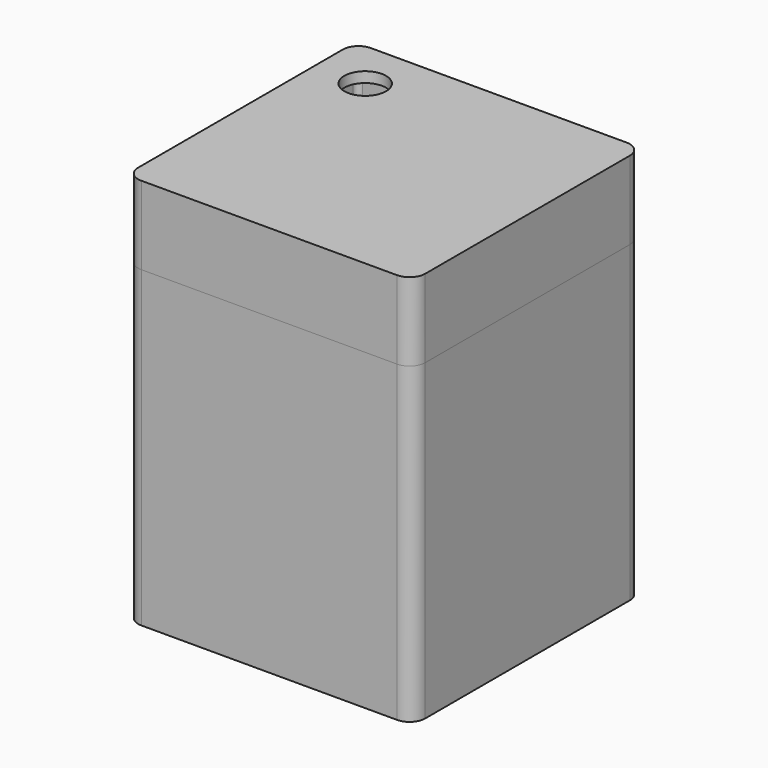
from build123d import *

# Parameters (mm, degrees)
F0_W      = 55
F0_H      = 55
F1_DEPTH  = 15
F2_R      = 3
F3_T      = -2
F4_R      = 4
F5_DEPTH  = 25
F6_DEPTH  = 60
F8_DEPTH  = 3
F9_W      = 5
F9_H      = 5
F10_DEPTH = 5
F11_R     = 2
F13_D     = 1.8
F13_DEPTH = 5
F13_TIP   = 0.5407745571


# Not quite as in the source:
# - a feature names something its author has since deleted; it is built from what else it names


with BuildPart() as f1:
    # F0 (on Top) → F1 (new body)
    with BuildSketch(Plane.XY):
        Rectangle(F0_W, F0_H)
    extrude(amount=F1_DEPTH)

    # F2
    f2_edges = [f1.edges().sort_by_distance(p)[0] for p in [
        (-27.5, 27.5, 7.5),
        (-27.5, -27.5, 7.5),
        (27.5, -27.5, 7.5),
        (27.5, 27.5, 7.5),
    ]]
    fillet(f2_edges, radius=F2_R)

    # F3
    f3_openings = [f1.faces().sort_by_distance(p)[0] for p in [
        (0, 0, 0),
    ]]
    offset(amount=F3_T, openings=f3_openings)

    # F4 (on face) → F5 (cut)
    with BuildSketch(Plane.XY.offset(15)):
        with Locations((-18, 18)):
            Circle(F4_R)
    extrude(amount=-F5_DEPTH, mode=Mode.SUBTRACT)


with BuildPart() as f6:
    # F6 (new): a face of the model
    f6_faces = [f1.part.faces().sort_by_distance(p)[0] for p in [
        (0, -26.7221825407, 0),
    ]]
    extrude(f6_faces, amount=F6_DEPTH)

    # F7 (on face) → F8 (cut)
    with BuildSketch(Plane(origin=(0, 0, -60), x_dir=(1, 0, 0), z_dir=(0, 0, -1))):
        with BuildLine():
            Line((-24.05, -26.55), (24.05, -26.55))
            ThreePointArc((24.05, -26.55), (25.817766953, -25.817766953), (26.55, -24.05))
            Line((26.55, -24.05), (26.55, 24.05))
            ThreePointArc((26.55, 24.05), (25.817766953, 25.817766953), (24.05, 26.55))
            Line((24.05, 26.55), (-24.05, 26.55))
            ThreePointArc((-24.05, 26.55), (-25.817766953, 25.817766953), (-26.55, 24.05))
            Line((-26.55, 24.05), (-26.55, -24.05))
            ThreePointArc((-26.55, -24.05), (-25.817766953, -25.817766953), (-24.05, -26.55))
        make_face()
    extrude(amount=-F8_DEPTH, mode=Mode.SUBTRACT)


with BuildPart() as f1_1:
    add(f1.part)

    # F9 (on face) → F10 (join)
    with BuildSketch(Plane(origin=(0, 0, 13), x_dir=(1, 0, 0), z_dir=(0, 0, -1))):
        with Locations((-23, 0)):
            Rectangle(F9_W, F9_H)
        with Locations((0, -23)):
            Rectangle(F9_W, F9_H)
        with Locations((0, 23)):
            Rectangle(F9_W, F9_H)
        with Locations((23, -5)):
            Rectangle(F9_W, F9_H)
    extrude(amount=F10_DEPTH)

    # F11
    f11_edges = [f1_1.edges().sort_by_distance(p)[0] for p in [
        (-20.5, 2.5, 10.5),
        (-20.5, -2.5, 10.5),
        (2.5, 20.5, 10.5),
        (-2.5, 20.5, 10.5),
        (-2.5, -20.5, 10.5),
        (2.5, -20.5, 10.5),
        (20.5, 2.5, 10.5),
        (20.5, 7.5, 10.5),
    ]]
    fillet(f11_edges, radius=F11_R)

    # F13
    with Locations(Plane(origin=(0, 0, 8), x_dir=(1, 0, 0), z_dir=(0, 0, -1))):
        with Locations((23, -5), (0, -23), (0, 23), (-23, 0)):
            Hole(F13_D / 2, depth=F13_DEPTH)
            with Locations((0, 0, -(F13_DEPTH + F13_TIP / 2))):  # 118° drill point
                Cone(0, F13_D / 2, F13_TIP, mode=Mode.SUBTRACT)


solid = Compound([f6.part, f1_1.part])
